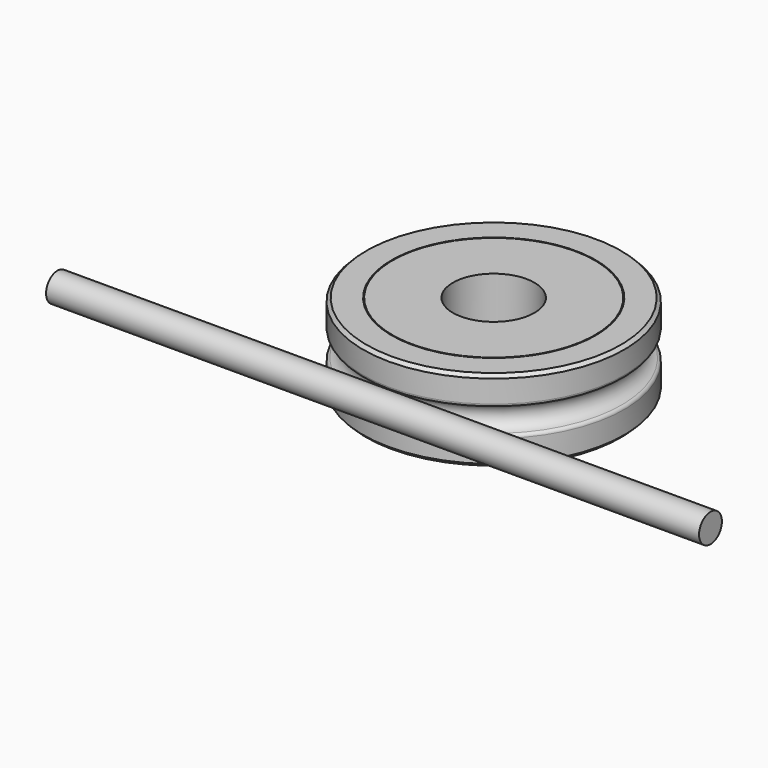
from build123d import *

# Parameters (mm, degrees)
F0_R     = 6.2
F0_R_2   = 2.5
F1_DEPTH = 5
F4_SIZE  = 0.2
F2_R     = 0.875
F5_DEPTH = 20
F6_ANGLE = 90


with BuildPart() as f1:
    # F0 (on Top) → F1 (new body)
    with BuildSketch(Plane.XY):
        Circle(F0_R)
        Circle(F0_R_2, mode=Mode.SUBTRACT)
    extrude(amount=F1_DEPTH)


with BuildPart() as f3:
    # F2 (on Front) → F3 (revolve)
    with BuildSketch(Plane.XZ):
        with BuildLine():
            Line((-8, 1.5712912189), (-8, 0))
            Line((-8, 0), (-6.25, 0))
            Line((-6.25, 0), (-6.25, 5))
            Line((-6.25, 5), (-8, 5))
            Line((-8, 5), (-8, 3.4287087811))
            ThreePointArc((-8, 3.4287087811), (-7.955597321, 3.3030526086), (-7.8421052632, 3.2331911429))
            ThreePointArc((-7.8421052632, 3.2331911429), (-7.25, 2.5), (-7.8421052632, 1.7668088571))
            ThreePointArc((-7.8421052632, 1.7668088571), (-7.955597321, 1.6969473914), (-8, 1.5712912189))
        make_face()
    revolve(axis=Axis((0, 0, 3.1425277703), (0, 0, 1)))

    # F4
    f4_edges = [f3.edges().sort_by_distance(p)[0] for p in [
        (8, 0, 0),
        (8, 0, 5),
    ]]
    chamfer(f4_edges, length=F4_SIZE)


with BuildPart() as f5:
    # F2 (on Front) → F5 (new body, symmetric)
    with BuildSketch(Plane.XZ):
        with Locations((-8.4, 2.5)):
            Circle(F2_R)
    extrude(amount=F5_DEPTH, both=True)


with BuildPart() as f1_1:
    # F6: moved
    add(f1.part.rotate(Axis((0, 0, 0), (0, 0, 1)), F6_ANGLE))


with BuildPart() as f3_1:
    # F6: moved
    add(f3.part.rotate(Axis((0, 0, 0), (0, 0, 1)), F6_ANGLE))


with BuildPart() as f5_1:
    # F6: moved
    add(f5.part.rotate(Axis((0, 0, 0), (0, 0, 1)), F6_ANGLE))


solid = Compound([f1_1.part, f3_1.part, f5_1.part])
